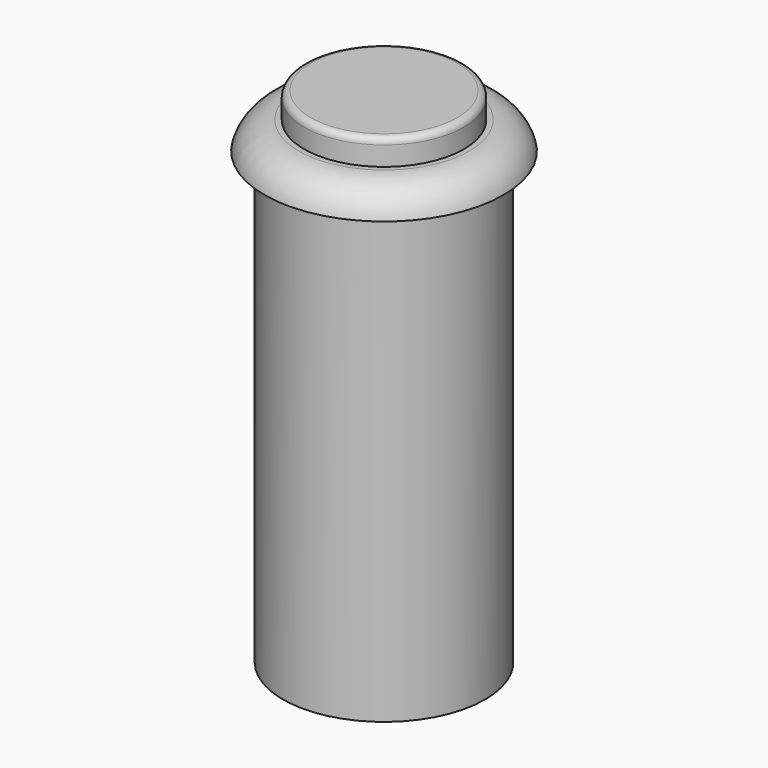
from build123d import *

# Parameters (mm, degrees)
F0_R     = 16.51
F0_R_2   = 11.049
F1_DEPTH = 3.81
F2_DEPTH = 7.366
F4_R     = 0.889
F5_R     = 13.97
F5_R_2   = 11.049
F6_DEPTH = 62.23


# Not quite as in the source:
# - a fillet or chamfer that OpenCascade refuses, or shapes differently, is made with other operations: its cross-section is extruded or revolved along the edge and cut away or added


with BuildPart() as f1:
    # F0 (on Top) → F1 (new body)
    with BuildSketch(Plane.XY):
        Circle(F0_R)
        Circle(F0_R_2, mode=Mode.SUBTRACT)
    extrude(amount=F1_DEPTH)

    # F0 (on Top) → F2 (join)
    with BuildSketch(Plane.XY):
        Circle(F0_R_2)
    extrude(amount=F2_DEPTH)

    # F3: fillet of radius 4.826 on 1 edges, made by hand

    # F3_s1 → F3_t2 (revolve, cut)
    with BuildSketch(Plane.XZ):
        with BuildLine():
            ThreePointArc((16.51, 0), (14.8242428344, 2.7385633568), (11.7921593923, 3.81))
            Line((11.7921593923, 3.81), (16.51, 3.81))
            Line((16.51, 3.81), (16.51, 0))
        make_face()
    revolve(axis=Axis((0, 0, 3.81), (0, 0, 1)), mode=Mode.SUBTRACT)

    # F4
    f4_edges = [f1.edges().sort_by_distance(p)[0] for p in [
        (-11.049, 0, 7.366),
    ]]
    fillet(f4_edges, radius=F4_R)

    # F5 (on face) → F6 (join)
    with BuildSketch(Plane.XY):
        Circle(F5_R)
        Circle(F5_R_2, mode=Mode.SUBTRACT)
        Circle(F5_R_2)
    extrude(amount=-F6_DEPTH)


solid = f1.part
